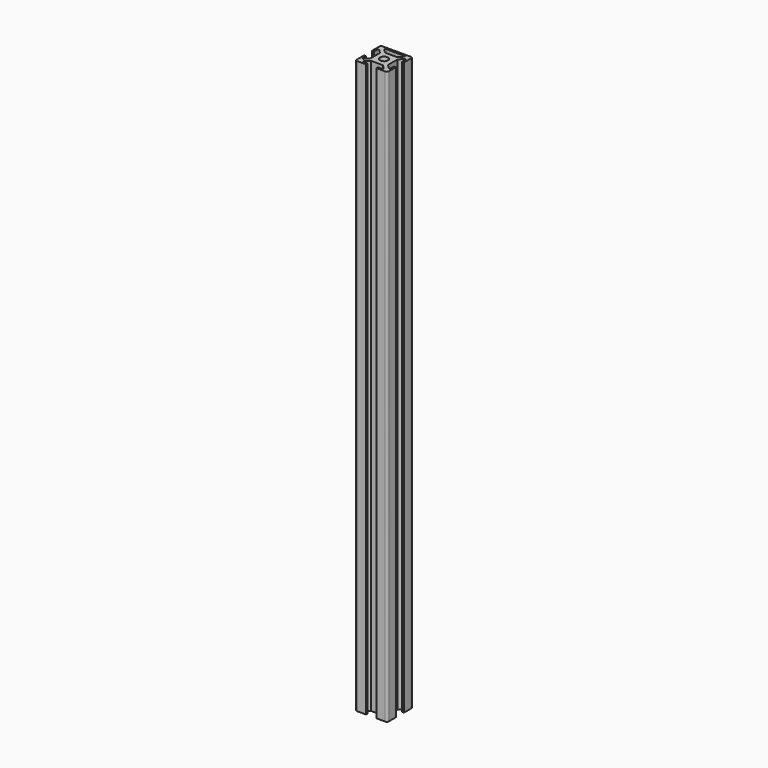
from build123d import *

# Parameters (mm, degrees)
F0_W        = 25.4
F0_H        = 25.4
F1_DEPTH    = 455.93
F3_DEPTH    = 455.93
F4_R        = 3.175
F5_DEPTH    = 455.93
F6_T1_DEPTH = 463.8675
F7_T1_DEPTH = 455.93
F8_W        = 8.2098719395
F8_H        = 1.5875
F9_DEPTH    = 455.93


# Not quite as in the source:
# - a fillet or chamfer that OpenCascade refuses, or shapes differently, is made with other operations: its cross-section is extruded or revolved along the edge and cut away or added


with BuildPart() as f1:
    # F0 (on Top) → F1 (new body)
    with BuildSketch(Plane.XY):
        Rectangle(F0_W, F0_H)
    extrude(amount=F1_DEPTH)

    # F2 (on face) → F3 (cut)
    with BuildSketch(Plane.XY.offset(455.93)):
        Polygon((-7.0075640303, -4.7625), (-7.0075640303, 4.7625), (-11.1125, 8.8674359697), (-11.1125, 4.1049359697), (-12.7, 4.1049359697), (-12.7, -4.1049359697), (-11.1125, -4.1049359697), (-11.1125, -8.8674359697), align=None)
        Polygon((4.1049359697, 12.7), (-4.1049359697, 12.7), (-4.1049359697, 11.1125), (-8.8674359697, 11.1125), (-4.7625, 7.0075640303), (4.7625, 7.0075640303), (8.8674359697, 11.1125), (4.1049359697, 11.1125), align=None)
        Polygon((12.7, -4.1049359697), (12.7, 4.1049359697), (11.1125, 4.1049359697), (11.1125, 8.8674359697), (7.0075640303, 4.7625), (7.0075640303, -4.7625), (11.1125, -8.8674359697), (11.1125, -4.1049359697), align=None)
        Polygon((-4.1049359697, -11.1125), (-4.1049359697, -12.7), (4.1049359697, -12.7), (4.1049359697, -11.1125), (8.8674359697, -11.1125), (4.7625, -7.0075640303), (-4.7625, -7.0075640303), (-8.8674359697, -11.1125), align=None)
    extrude(amount=-F3_DEPTH, mode=Mode.SUBTRACT)

    # F4 (on face) → F5 (cut)
    with BuildSketch(Plane.XY.offset(455.93)):
        Circle(F4_R)
    extrude(amount=-F5_DEPTH, mode=Mode.SUBTRACT)

    # F6: fillet of radius 1.5875 on 4 edges, made by hand

    # F6_s2 → F6_t1 (cut)
    with BuildSketch(Plane.XY.offset(-3.96875)):
        with BuildLine():
            add(Edge.make_bspline(
                [(-12.7, 11.1125), (-12.7, 12.7), (-11.1125, 12.7)],
                knots=[0, 0, 0, 1, 1, 1], degree=2, weights=[1, 1, 1]))
            Line((-11.1125, 12.7), (-12.7, 12.7))
            Line((-12.7, 12.7), (-12.7, 11.1125))
        make_face()
        with BuildLine():
            add(Edge.make_bspline(
                [(12.7, 11.1125), (12.7, 12.7), (11.1125, 12.7)],
                knots=[0, 0, 0, 1, 1, 1], degree=2, weights=[1, 1, 1]))
            Line((11.1125, 12.7), (12.7, 12.7))
            Line((12.7, 12.7), (12.7, 11.1125))
        make_face()
        with BuildLine():
            add(Edge.make_bspline(
                [(12.7, -11.1125), (12.7, -12.7), (11.1125, -12.7)],
                knots=[0, 0, 0, 1, 1, 1], degree=2, weights=[1, 1, 1]))
            Line((11.1125, -12.7), (12.7, -12.7))
            Line((12.7, -12.7), (12.7, -11.1125))
        make_face()
        with BuildLine():
            add(Edge.make_bspline(
                [(-11.1125, -12.7), (-12.7, -12.7), (-12.7, -11.1125)],
                knots=[0, 0, 0, 1, 1, 1], degree=2, weights=[1, 1, 1]))
            Line((-12.7, -11.1125), (-12.7, -12.7))
            Line((-12.7, -12.7), (-11.1125, -12.7))
        make_face()
    extrude(amount=F6_T1_DEPTH, mode=Mode.SUBTRACT)

    # F7: fillet of radius 0.79375 on 8 edges, made by hand

    # F7_s2 → F7_t1 (join)
    with BuildSketch(Plane.XY):
        with BuildLine():
            add(Edge.make_bspline(
                [(-9.7574839924, 7.5124199622), (-11.1125, 8.8674359697), (-11.1125, 6.9511539546)],
                knots=[0, 0, 0, 1, 1, 1], degree=2, weights=[1, 1, 1]))
            Line((-11.1125, 6.9511539546), (-11.1125, 8.8674359697))
            Line((-11.1125, 8.8674359697), (-9.7574839924, 7.5124199622))
        make_face()
        with BuildLine():
            add(Edge.make_bspline(
                [(11.1125, 6.9511539546), (11.1125, 8.8674359697), (9.7574839924, 7.5124199622)],
                knots=[0, 0, 0, 1, 1, 1], degree=2, weights=[1, 1, 1]))
            Line((9.7574839924, 7.5124199622), (11.1125, 8.8674359697))
            Line((11.1125, 8.8674359697), (11.1125, 6.9511539546))
        make_face()
        with BuildLine():
            add(Edge.make_bspline(
                [(9.7574839924, -7.5124199622), (11.1125, -8.8674359697), (11.1125, -6.9511539546)],
                knots=[0, 0, 0, 1, 1, 1], degree=2, weights=[1, 1, 1]))
            Line((11.1125, -6.9511539546), (11.1125, -8.8674359697))
            Line((11.1125, -8.8674359697), (9.7574839924, -7.5124199622))
        make_face()
        with BuildLine():
            add(Edge.make_bspline(
                [(-11.1125, -6.9511539546), (-11.1125, -8.8674359697), (-9.7574839924, -7.5124199622)],
                knots=[0, 0, 0, 1, 1, 1], degree=2, weights=[1, 1, 1]))
            Line((-9.7574839924, -7.5124199622), (-11.1125, -8.8674359697))
            Line((-11.1125, -8.8674359697), (-11.1125, -6.9511539546))
        make_face()
        with BuildLine():
            add(Edge.make_bspline(
                [(-7.5124199622, -9.7574839924), (-8.8674359697, -11.1125), (-6.9511539546, -11.1125)],
                knots=[0, 0, 0, 1, 1, 1], degree=2, weights=[1, 1, 1]))
            Line((-6.9511539546, -11.1125), (-8.8674359697, -11.1125))
            Line((-8.8674359697, -11.1125), (-7.5124199622, -9.7574839924))
        make_face()
        with BuildLine():
            add(Edge.make_bspline(
                [(6.9511539546, -11.1125), (8.8674359697, -11.1125), (7.5124199622, -9.7574839924)],
                knots=[0, 0, 0, 1, 1, 1], degree=2, weights=[1, 1, 1]))
            Line((7.5124199622, -9.7574839924), (8.8674359697, -11.1125))
            Line((8.8674359697, -11.1125), (6.9511539546, -11.1125))
        make_face()
        with BuildLine():
            add(Edge.make_bspline(
                [(7.5124199622, 9.7574839924), (8.8674359697, 11.1125), (6.9511539546, 11.1125)],
                knots=[0, 0, 0, 1, 1, 1], degree=2, weights=[1, 1, 1]))
            Line((6.9511539546, 11.1125), (8.8674359697, 11.1125))
            Line((8.8674359697, 11.1125), (7.5124199622, 9.7574839924))
        make_face()
        with BuildLine():
            add(Edge.make_bspline(
                [(-6.9511539546, 11.1125), (-8.8674359697, 11.1125), (-7.5124199622, 9.7574839924)],
                knots=[0, 0, 0, 1, 1, 1], degree=2, weights=[1, 1, 1]))
            Line((-7.5124199622, 9.7574839924), (-8.8674359697, 11.1125))
            Line((-8.8674359697, 11.1125), (-6.9511539546, 11.1125))
        make_face()
    extrude(amount=F7_T1_DEPTH)

    # F8 (on face) → F9 (join)
    with BuildSketch(Plane.XY.offset(455.93)):
        with Locations((0, 11.90625)):
            Rectangle(F8_W, F8_H)
    extrude(amount=-F9_DEPTH)


solid = f1.part
